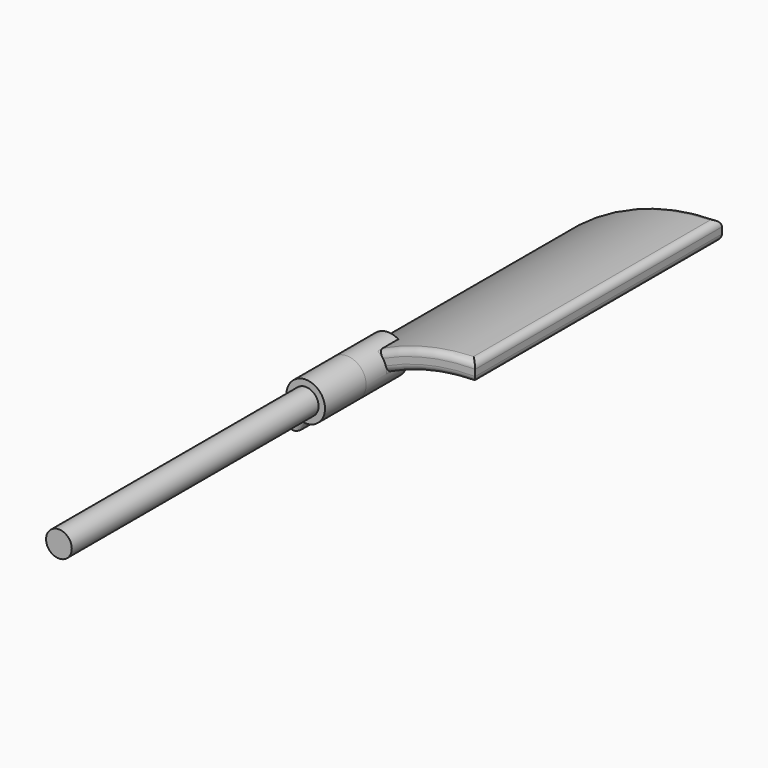
from build123d import *

# Parameters (mm, degrees)
F1_DEPTH     = 76.2
F2_R         = 4.7625
F3_DEPTH     = 6.35
F4_R         = 4.7625
F5_DEPTH     = 12.7
F6_R         = 3.175
F7_DEPTH     = 76.2
F8_T1_DEPTH  = 84.4391678442
F8_T3_DEPTH  = 84.0788040297
F8_T8_ANGLE  = 33.9025331494
F8_S9_R      = 4.7625
F8_T10_DEPTH = 21
F8_T14_ANGLE = 34.4766821812
F8_S15_R     = 4.7625
F8_T16_DEPTH = 21
F8_T20_ANGLE = 33.9025331494
F8_S21_R     = 4.7625
F8_T22_DEPTH = 20
F8_T26_ANGLE = 34.4766821812
F8_S27_R     = 4.7625
F8_T28_DEPTH = 20
F8_T30_ANGLE = 68.2520650555
F8_T32_ANGLE = 69.0256961544


# Not quite as in the source:
# - a fillet or chamfer that OpenCascade refuses, or shapes differently, is made with other operations: its cross-section is extruded or revolved along the edge and cut away or added


with BuildPart() as f1:
    # F0 (on Front) → F1 (new body)
    with BuildSketch(Plane.XZ):
        with BuildLine():
            Line((0, 50.8), (0, 55.5625))
            ThreePointArc((0, 55.5625), (-27.78125, 48.1185364978), (-48.1185364978, 27.78125))
            Line((-48.1185364978, 27.78125), (-43.9940905122, 25.4))
            ThreePointArc((-43.9940905122, 25.4), (-25.4, 43.9940905122), (0, 50.8))
        make_face()
    extrude(amount=F1_DEPTH)

    # F2 (on face) → F3 (join, symmetric)
    with BuildSketch(Plane.XZ.offset(76.2)):
        with Locations((-26.590625, 46.056313505)):
            Circle(F2_R)
    extrude(amount=F3_DEPTH, both=True)

    # F4 (on face) → F5 (join)
    with BuildSketch(Plane.XZ.offset(82.55)):
        with Locations((-26.590625, 46.056313505)):
            Circle(F4_R)
    extrude(amount=F5_DEPTH)

    # F6 (on face) → F7 (join)
    with BuildSketch(Plane.XZ.offset(95.25)):
        with Locations((-26.590625, 46.056313505)):
            Circle(F6_R)
    extrude(amount=F7_DEPTH)

    # F8: fillet of radius 1.6002 on 10 edges, made by hand

    # F8_s2 → F8_t1 (cut)
    with BuildSketch(Plane.XZ.offset(-4.1195839221)):
        with BuildLine():
            ThreePointArc((-46.7121706404, 26.9692842937), (-47.4637166662, 27.9639017102), (-47.2735488472, 29.1959412529))
            ThreePointArc((-47.2735488472, 29.1959412529), (-47.7012874507, 28.4917283049), (-48.1185364978, 27.78125))
            Line((-48.1185364978, 27.78125), (-46.7121706404, 26.9692842937))
        make_face()
        with BuildLine():
            ThreePointArc((-1.6476523888, 55.5380648552), (-0.4855909368, 55.0867352461), (0, 53.9385685873))
            Line((0, 53.9385685873), (0, 55.5625))
            ThreePointArc((0, 55.5625), (-0.8239167844, 55.5563908779), (-1.6476523888, 55.5380648552))
        make_face()
    extrude(amount=F8_T1_DEPTH, mode=Mode.SUBTRACT)

    # F8_s4 → F8_t3 (cut)
    with BuildSketch(Plane.XZ.offset(-3.9394020148)):
        with BuildLine():
            ThreePointArc((-45.3587394005, 26.187880403), (-44.1681291542, 26.0218753898), (-43.197905381, 26.7316473622))
            ThreePointArc((-43.197905381, 26.7316473622), (-43.6010820753, 26.0688634556), (-43.9940905122, 25.4))
            Line((-43.9940905122, 25.4), (-45.3587394005, 26.187880403))
        make_face()
        with BuildLine():
            ThreePointArc((-1.5513330102, 50.7763071313), (-0.4515405646, 51.2616595801), (0, 52.3757608059))
            Line((0, 52.3757608059), (0, 50.8))
            ThreePointArc((0, 50.8), (-0.7757569627, 50.7940764375), (-1.5513330102, 50.7763071313))
        make_face()
    extrude(amount=F8_T3_DEPTH, mode=Mode.SUBTRACT)


with BuildPart() as f8_tool6:
    # F8_s7 → F8_t8 (revolve)
    with BuildSketch(Plane(origin=(0, 0, 0), x_dir=(0, 1, 0), z_dir=(0.8640737071, 0, 0.5033653034))):
        with BuildLine():
            ThreePointArc((-74.5998, 55.5625), (-75.7313122713, 55.0938122713), (-76.2, 53.9623))
            Line((-76.2, 53.9623), (-76.2, 55.5625))
            Line((-76.2, 55.5625), (-74.5998, 55.5625))
        make_face()
    revolve(axis=Axis((0, -76.2, 0), (0, -1, 0)), revolution_arc=F8_T8_ANGLE)

    # F8_s9 → F8_t10 (cut, symmetric)
    with BuildSketch(Plane.XZ.offset(75.4)):
        with Locations((-26.590625, 46.056313505)):
            Circle(F8_S9_R)
    extrude(amount=F8_T10_DEPTH, both=True, mode=Mode.SUBTRACT)


with BuildPart() as f1_1:
    add(f1.part)

    # F8_t5: cut F8_tool6
    add(f8_tool6.part, mode=Mode.SUBTRACT)


with BuildPart() as f8_tool12:
    # F8_s13 → F8_t14 (revolve)
    with BuildSketch(Plane(origin=(0, 0, 0), x_dir=(0, 1, 0), z_dir=(-0.4303190954, 0, -0.9026768393))):
        with BuildLine():
            ThreePointArc((-74.5998, -50.8), (-75.7313122713, -51.2686877287), (-76.2, -52.4002))
            Line((-76.2, -52.4002), (-76.2, -50.8))
            Line((-76.2, -50.8), (-74.5998, -50.8))
        make_face()
    revolve(axis=Axis((0, -76.2, 0), (0, 1, 0)), revolution_arc=F8_T14_ANGLE)

    # F8_s15 → F8_t16 (cut, symmetric)
    with BuildSketch(Plane.XZ.offset(74.8)):
        with Locations((-26.590625, 46.056313505)):
            Circle(F8_S15_R)
    extrude(amount=F8_T16_DEPTH, both=True, mode=Mode.SUBTRACT)


with BuildPart() as f1_2:
    add(f1_1.part)

    # F8_t11: cut F8_tool12
    add(f8_tool12.part, mode=Mode.SUBTRACT)


with BuildPart() as f8_tool18:
    # F8_s19 → F8_t20 (revolve)
    with BuildSketch(Plane(origin=(0, 0, 0), x_dir=(0, 1, 0), z_dir=(0.9974089506, 0, -0.071940151))):
        with BuildLine():
            ThreePointArc((-74.5998, 55.5625), (-75.7313122713, 55.0938122713), (-76.2, 53.9623))
            Line((-76.2, 53.9623), (-76.2, 55.5625))
            Line((-76.2, 55.5625), (-74.5998, 55.5625))
        make_face()
    revolve(axis=Axis((0, -76.2, 0), (0, -1, 0)), revolution_arc=F8_T20_ANGLE)

    # F8_s21 → F8_t22 (cut, symmetric)
    with BuildSketch(Plane.XZ.offset(75.4)):
        with Locations((-26.590625, 46.056313505)):
            Circle(F8_S21_R)
    extrude(amount=F8_T22_DEPTH, both=True, mode=Mode.SUBTRACT)


with BuildPart() as f1_3:
    add(f1_2.part)

    # F8_t17: cut F8_tool18
    add(f8_tool18.part, mode=Mode.SUBTRACT)


with BuildPart() as f8_tool24:
    # F8_s25 → F8_t26 (revolve)
    with BuildSketch(Plane(origin=(0, 0, 0), x_dir=(0, 1, 0), z_dir=(-0.8663350804, 0, -0.4994632404))):
        with BuildLine():
            ThreePointArc((-74.5998, -50.8), (-75.7313122713, -51.2686877287), (-76.2, -52.4002))
            Line((-76.2, -52.4002), (-76.2, -50.8))
            Line((-76.2, -50.8), (-74.5998, -50.8))
        make_face()
    revolve(axis=Axis((0, -76.2, 0), (0, 1, 0)), revolution_arc=F8_T26_ANGLE)

    # F8_s27 → F8_t28 (cut, symmetric)
    with BuildSketch(Plane.XZ.offset(74.8)):
        with Locations((-26.590625, 46.056313505)):
            Circle(F8_S27_R)
    extrude(amount=F8_T28_DEPTH, both=True, mode=Mode.SUBTRACT)


with BuildPart() as f1_4:
    add(f1_3.part)

    # F8_t23: cut F8_tool24
    add(f8_tool24.part, mode=Mode.SUBTRACT)

    # F8_s29 → F8_t30 (revolve, cut)
    with BuildSketch(Plane(origin=(0, 0, 0), x_dir=(0, 1, 0), z_dir=(0.9974081949, 0, -0.0719506275))):
        with BuildLine():
            ThreePointArc((-1.6002, 55.5625), (-0.4686877287, 55.0938122713), (0, 53.9623))
            Line((0, 53.9623), (0, 55.5625))
            Line((0, 55.5625), (-1.6002, 55.5625))
        make_face()
    revolve(axis=Axis((0, 0, 0), (0, -1, 0)), revolution_arc=F8_T30_ANGLE, mode=Mode.SUBTRACT)

    # F8_s31 → F8_t32 (revolve, cut)
    with BuildSketch(Plane(origin=(0, 0, 0), x_dir=(0, 1, 0), z_dir=(-0.4303086891, 0, -0.9026818))):
        with BuildLine():
            ThreePointArc((-1.6002, -50.8), (-0.4686877287, -51.2686877287), (0, -52.4002))
            Line((0, -52.4002), (0, -50.8))
            Line((0, -50.8), (-1.6002, -50.8))
        make_face()
    revolve(axis=Axis((0, 0, 0), (0, 1, 0)), revolution_arc=F8_T32_ANGLE, mode=Mode.SUBTRACT)


solid = f1_4.part
